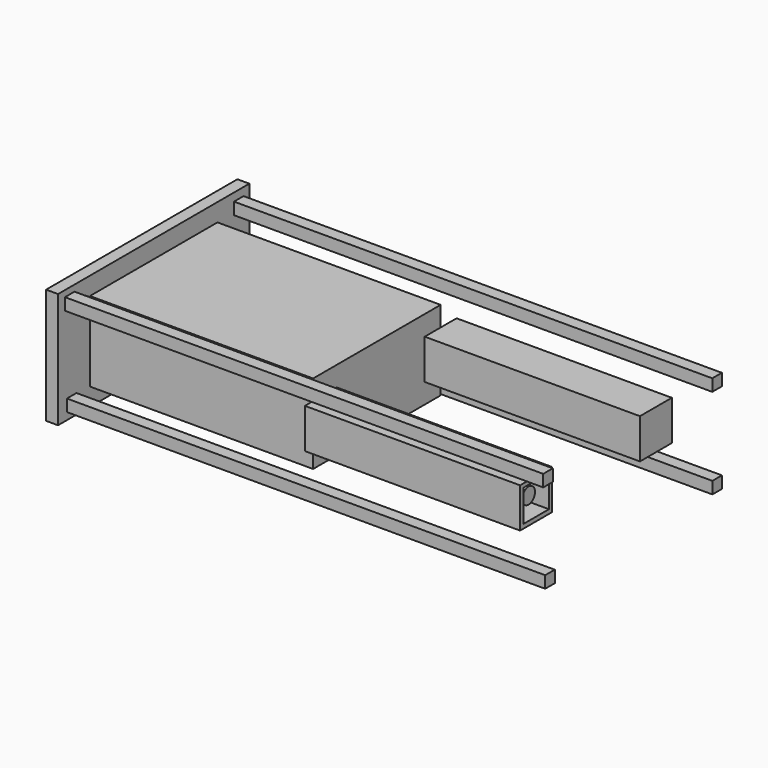
from build123d import *

# Parameters (mm, degrees)
F0_W      = 508
F0_H      = 254
F1_DEPTH  = 711.2
F2_W      = 482.6
F2_H      = 228.6
F3_DEPTH  = 685.8
F4_R      = 25.4
F5_DEPTH  = 660.4
F6_W      = 32.7536183119
F6_H      = 127
F6_W_2    = 94.2463816881
F7_DEPTH  = 685.8
F8_W      = 101.6
F8_H      = 101.6
F9_DEPTH  = 685.8
F10_R     = 25.4
F11_DEPTH = 660.4
F12_W     = 762
F12_H     = 368.1078273856
F13_DEPTH = 38.1
F14_W     = 63.5
F14_H     = 127
F15_DEPTH = 685.8
F16_W     = 101.6
F16_H     = 101.6
F17_DEPTH = 660.4
F18_R     = 25.4
F19_DEPTH = 660.4
F20_W     = 38.1
F20_H     = 38.1
F21_DEPTH = 1524
F22_R     = 25.4
F23_DEPTH = 660.4


with BuildPart() as f1:
    # F0 (on Right) → F1 (new body)
    with BuildSketch(Plane.YZ):
        Rectangle(F0_W, F0_H)
    extrude(amount=F1_DEPTH)

    # F2 (on face) → F3 (cut)
    with BuildSketch(Plane(origin=(0, 0, 0), x_dir=(0, -1, 0), z_dir=(-1, 0, 0))):
        Rectangle(F2_W, F2_H)
    extrude(amount=-F3_DEPTH, mode=Mode.SUBTRACT)

    # F6 (on face) → F7 (join)
    with BuildSketch(Plane.YZ.offset(711.2)):
        with Locations((-270.3768091559, 0)):
            Rectangle(F6_W, F6_H)
        with Locations((-206.8768091559, 0)):
            Rectangle(F6_W_2, F6_H)
    extrude(amount=F7_DEPTH)

    # F8 (on face) → F9 (cut)
    with BuildSketch(Plane.YZ.offset(711.2)):
        with Locations((-222.696326673, 0.6148855095)):
            Rectangle(F8_W, F8_H)
    extrude(amount=F9_DEPTH, mode=Mode.SUBTRACT)

    # F14 (on face) → F15 (join)
    with BuildSketch(Plane.YZ.offset(711.2)):
        with Locations((222.25, 0)):
            Rectangle(F14_W, F14_H)
        with Locations((285.75, 0)):
            Rectangle(F14_W, F14_H)
    extrude(amount=F15_DEPTH)

    # F16 (on face) → F17 (cut)
    with BuildSketch(Plane.YZ.offset(711.2)):
        with Locations((254.5926607187, 0)):
            Rectangle(F16_W, F16_H)
    extrude(amount=F17_DEPTH, mode=Mode.SUBTRACT)


with BuildPart() as f5:
    # F4 (on Right) → F5 (new body)
    with BuildSketch(Plane.YZ):
        Circle(F4_R)
    extrude(amount=F5_DEPTH)


with BuildPart() as f11:
    # F10 (on face) → F11 (new body)
    with BuildSketch(Plane.YZ.offset(711.2)):
        with Locations((-221.2180942297, 0)):
            Circle(F10_R)
    extrude(amount=F11_DEPTH)


with BuildPart() as f13:
    # F12 (on Right) → F13 (new body)
    with BuildSketch(Plane.YZ):
        Rectangle(F12_W, F12_H)
    extrude(amount=-F13_DEPTH)

    # F20 (on face) → F21 (join)
    with BuildSketch(Plane.YZ):
        with Locations((339.2434695244, -148.4175494432)):
            Rectangle(F20_W, F20_H)
        with Locations((338.8835170746, 139.4650766134)):
            Rectangle(F20_W, F20_H)
        with Locations((-334.4604074955, 145.0996161673)):
            Rectangle(F20_W, F20_H)
        with Locations((-326.5745958805, -142.3655322313)):
            Rectangle(F20_W, F20_H)
    extrude(amount=F21_DEPTH)


with BuildPart() as f19:
    # F18 (on face) → F19 (new body)
    with BuildSketch(Plane.YZ.offset(711.2)):
        with Locations((257.2414875031, 0)):
            Circle(F18_R)
    extrude(amount=F19_DEPTH)


with BuildPart() as f23:
    # F22 (on face) → F23 (new body)
    with BuildSketch(Plane.YZ):
        with Locations((-282.360881567, 112.1070384979)):
            Circle(F22_R)
    extrude(amount=F23_DEPTH)


with BuildPart() as f23b:
    # F22 (on face) → F23, piece 2 (new body)
    with BuildSketch(Plane.YZ):
        with Locations((285.1519286633, -122.3408728838)):
            Circle(F22_R)
    extrude(amount=F23_DEPTH)


solid = Compound([f1.part, f5.part, f11.part, f13.part, f19.part, f23.part, f23b.part])
